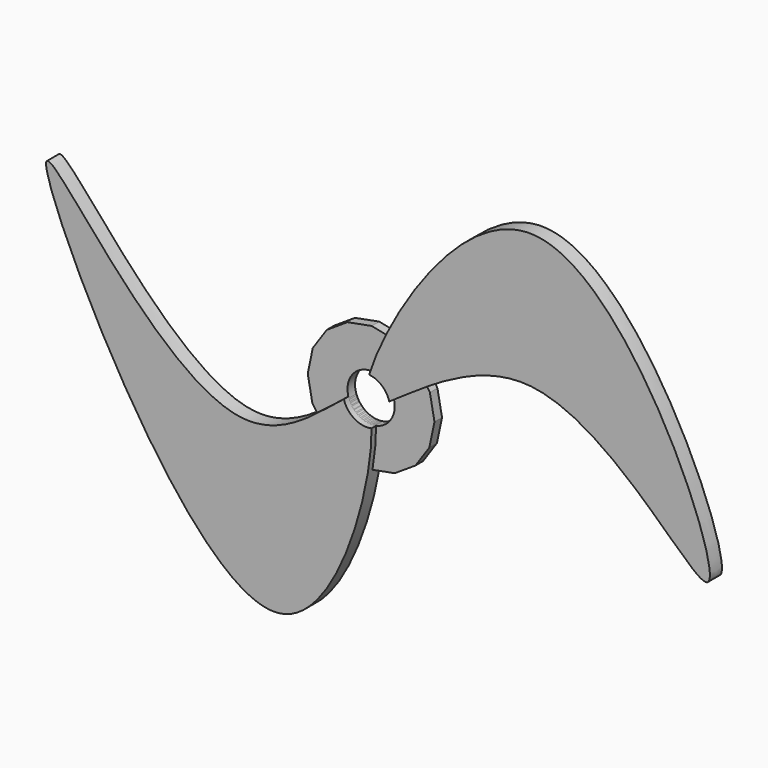
from build123d import *

# Parameters (mm, degrees)
F2_DEPTH = 2.032
F5_DEPTH = 1.27
F7_D     = 6.35
F7_2_D   = 6.35
F7_3_D   = 6.35


# Not quite as in the source:
# - the program builds the solid bodies; features that only make, move or delete a surface that nothing else refers to are left out


with BuildPart() as f2:
    # F1 (on Front) → F2 (new body)
    with BuildSketch(Plane.XZ):
        with BuildLine():
            add(Edge.make_bspline(
                [(0, 0), (-1.478108938, 2.9385077258), (23.5102189712, 54.0757384866), (58.3090351994, -28.8064935303), (23.1389765698, 22.7157851976), (1.7839165292, -1.7462149518), (0.1218154658, -0.1677448348)],
                knots=[0, 0, 0, 0, 0.262643161, 0.5467371715, 0.7845331571, 0.9940167235, 0.9940167235, 0.9940167235, 0.9940167235], degree=3))
            add(Edge.make_bspline(
                [(0, 0), (0.0426942227, -0.0499648339), (0.0832942879, -0.1059491623), (0.1218154658, -0.1677448348)],
                knots=[0, 0, 0, 0, 0.003989714, 0.003989714, 0.003989714, 0.003989714], degree=3))
        make_face()
    extrude(amount=F2_DEPTH)

    # F7 (through all)
    with Locations(Plane(origin=(0, 0, 0), x_dir=(1, 0, 0), z_dir=(0, 1, 0))):
        with Locations((0, 0)):
            Hole(F7_D / 2)


with BuildPart() as f2b:
    # F1 (on Front) → F2, piece 2 (new body)
    with BuildSketch(Plane.XZ):
        with BuildLine():
            add(Edge.make_bspline(
                [(0.1218154658, -0.1677448348), (0.0743424806, -0.1226605194), (0.0336728147, -0.0669421743), (0, 0)],
                knots=[0.9940167235, 0.9940167235, 0.9940167235, 0.9940167235, 1, 1, 1, 1], degree=3))
            add(Edge.make_bspline(
                [(0.1218154658, -0.1677448348), (2.4351202061, -3.8787482406), (-9.6021342591, -61.1609144488), (-60.037679205, 44.8368415658), (-17.435923871, -23.0492034133), (-1.9876053053, 2.3260844835), (0, 0)],
                knots=[0.003989714, 0.003989714, 0.003989714, 0.003989714, 0.2435832259, 0.5603402805, 0.8142611296, 1, 1, 1, 1], degree=3))
        make_face()
    extrude(amount=F2_DEPTH)

    # F7#2 (through all)
    with Locations(Plane(origin=(0, 0, 0), x_dir=(1, 0, 0), z_dir=(0, 1, 0))):
        with Locations((0, 0)):
            Hole(F7_2_D / 2)


with BuildPart() as f5:
    # F4 (on Front) → F5 (new body)
    with BuildSketch(Plane.XZ):
        Polygon((7.9152016549, 3.1864661835), (6.0932849885, 5.9729274251), (3.3437209183, 7.850064611), (0.0851056492, 8.5321006209), (-3.1864661835, 7.9152016549), (-5.9729274251, 6.0932849885), (-7.850064611, 3.3437209183), (-8.5321006209, 0.0851056492), (-7.9152016549, -3.1864661835), (-6.0932849885, -5.9729274251), (-3.3437209183, -7.850064611), (-0.0851056492, -8.5321006209), (3.1864661835, -7.9152016549), (5.9729274251, -6.0932849885), (7.850064611, -3.3437209183), (8.5321006209, -0.0851056492), align=None)
    extrude(amount=F5_DEPTH)

    # F7#3 (through all)
    with Locations(Plane(origin=(0, 0, 0), x_dir=(1, 0, 0), z_dir=(0, 1, 0))):
        with Locations((0, 0)):
            Hole(F7_3_D / 2)


solid = Compound([f2.part, f2b.part, f5.part])
